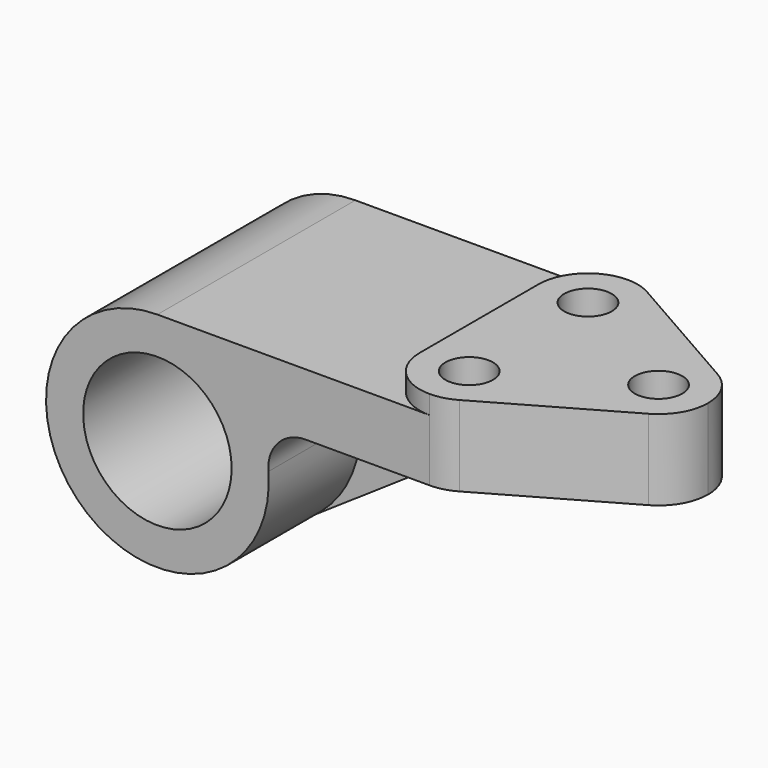
from build123d import *

# Parameters (mm, degrees)
F0_R          = 19.05
F1_DEPTH      = 63.5
F3_DEPTH      = 15.875
F3_DEPTH_BACK = 4.7752
F4_R          = 6.096
F5_DEPTH      = 61.9262
F8_DEPTH      = 2.38125


with BuildPart() as f1:
    # F0 (on Front) → F1 (new body)
    with BuildSketch(Plane.XZ):
        with BuildLine():
            Line((69.85, 28.575), (0, 28.575))
            ThreePointArc((0, 28.575), (-19.345366451, -21.0306305629), (28.4756083945, 2.38125))
            ThreePointArc((28.4756083945, 2.38125), (30.9572676717, 9.6234554837), (37.9674778593, 12.7))
            Line((37.9674778593, 12.7), (69.85, 12.7))
            Line((69.85, 12.7), (69.85, 28.575))
        make_face()
        Circle(F0_R, mode=Mode.SUBTRACT)
    extrude(amount=F1_DEPTH)

    # F2 (on face) → F3 (join, two sides)
    with BuildSketch(Plane.XY.offset(28.575)) as f3_sk:
        with BuildLine():
            ThreePointArc((76.1491554441, -1.6722785358), (73.1086759125, -0.4251871176), (69.85, 0))
            ThreePointArc((69.85, 0), (60.8697438789, -3.7197438789), (57.15, -12.7))
            Line((57.15, -12.7), (57.15, -31.75))
            Line((57.15, -31.75), (57.15, -50.8))
            ThreePointArc((57.15, -50.8), (60.8697438789, -59.7802561211), (69.85, -63.5))
            ThreePointArc((69.85, -63.5), (73.1086759125, -63.0748128824), (76.1491554441, -61.8277214642))
            Line((76.1491554441, -61.8277214642), (109.4993554441, -42.7777214642))
            ThreePointArc((109.4993554441, -42.7777214642), (114.1840352623, -38.1253715915), (115.9002, -31.75))
            ThreePointArc((115.9002, -31.75), (114.1840352623, -25.3746284085), (109.4993554441, -20.7222785358))
            Line((109.4993554441, -20.7222785358), (76.1491554441, -1.6722785358))
        make_face()
    extrude(amount=-F3_DEPTH)
    extrude(f3_sk.sketch, amount=F3_DEPTH_BACK)

    # F4 (on face) → F5 (cut, through all)
    with BuildSketch(Plane.XY.offset(33.3502)):
        with Locations((69.85, -12.7)):
            Circle(F4_R)
        with Locations((69.85, -50.8)):
            Circle(F4_R)
        with Locations((103.2002, -31.75)):
            Circle(F4_R)
    extrude(amount=-F5_DEPTH, mode=Mode.SUBTRACT)

    # F7 (on offset) → F8 (join, symmetric)
    with BuildSketch(Plane.XZ.offset(31.75)):
        with BuildLine():
            ThreePointArc((28.4756083945, 2.38125), (25.7719232537, -12.3425522809), (15.9950252975, -23.6788891364))
            Line((15.9950252975, -23.6788891364), (69.85, 12.7))
            Line((69.85, 12.7), (37.9674778593, 12.7))
            ThreePointArc((37.9674778593, 12.7), (30.9572676717, 9.6234554837), (28.4756083945, 2.38125))
        make_face()
    extrude(amount=F8_DEPTH, both=True)


solid = f1.part
